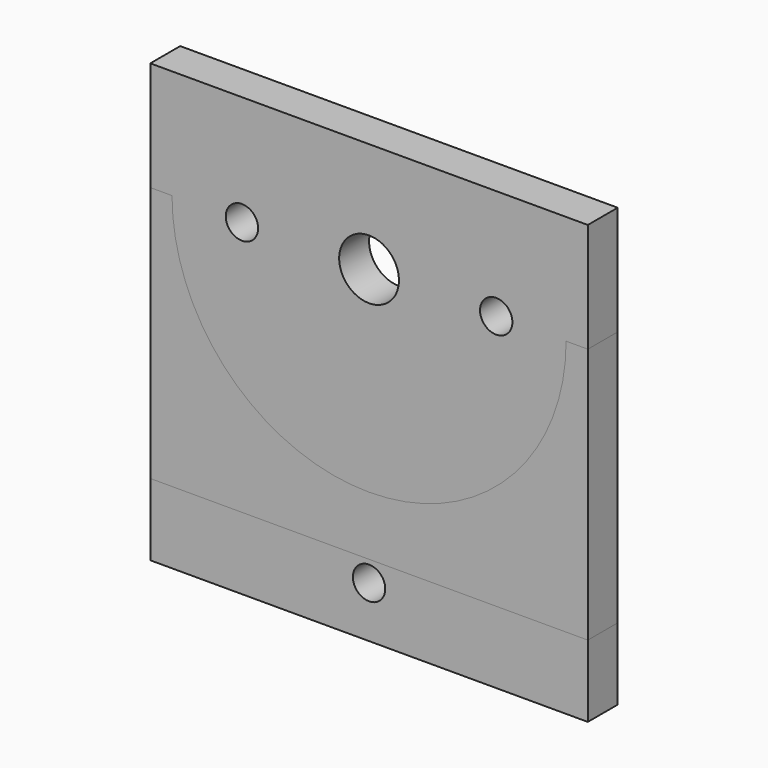
from build123d import *

# Parameters (mm, degrees)
F0_W     = 35.138
F0_H     = 35.138
F0_R     = 1.3
F0_R_2   = 2.4
F1_DEPTH = 3
F3_DEPTH = 3
F4_R     = 15.825
F5_DEPTH = 25


with BuildPart() as f1:
    # F0 (on Front) → F1 (new body)
    with BuildSketch(Plane.XZ):
        Rectangle(F0_W, F0_H)
        with Locations((0, -13.45565)):
            Circle(F0_R, mode=Mode.SUBTRACT)
        with Locations((-10.2108, 8.71855)):
            Circle(F0_R, mode=Mode.SUBTRACT)
        with Locations((0, 8.71855)):
            Circle(F0_R_2, mode=Mode.SUBTRACT)
        with Locations((10.2108, 8.71855)):
            Circle(F0_R, mode=Mode.SUBTRACT)
    extrude(amount=F1_DEPTH)


with BuildPart() as f3:
    # F2 (on Front) → F3 (new body)
    with BuildSketch(Plane.XZ):
        Polygon((17.569, 8.7845), (-17.569, 8.7845), (-17.569, -8.7845), (-17.569, -11.7845), (17.569, -11.7845), (17.569, -8.7845), align=None)
    extrude(amount=F3_DEPTH)

    # F4 (on face) → F5 (cut)
    with BuildSketch(Plane.XZ.offset(3)):
        with Locations((0, 8.7845)):
            Circle(F4_R)
    extrude(amount=-F5_DEPTH, mode=Mode.SUBTRACT)


solid = Compound([f1.part, f3.part])
